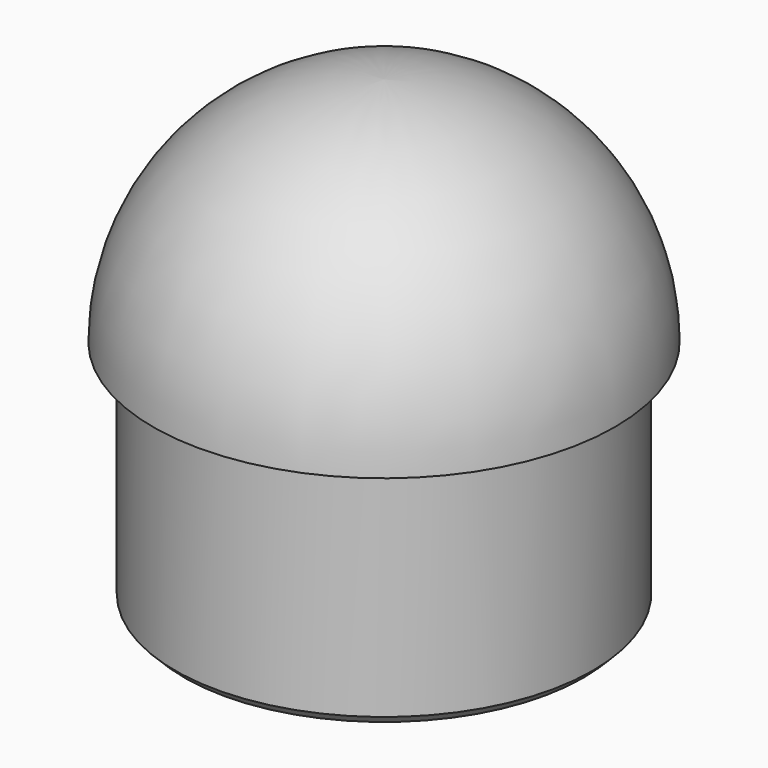
from build123d import *

# Parameters (mm, degrees)
F0_R     = 12.5
F1_DEPTH = 12.5
F2_R     = 12.49999
F3_R     = 11.3
F4_DEPTH = 12.5
F5_SIZE  = 0.5


# Not quite as in the source:
# - a fillet or chamfer is up to 0.001 mm smaller than in the source, because OpenCascade refuses the exact size


with BuildPart() as f1:
    # F0 (on Top) → F1 (new body)
    with BuildSketch(Plane.XY):
        Circle(F0_R)
    extrude(amount=F1_DEPTH)

    # F2 (radius 12.5 in the source; OpenCascade refuses exactly that, so slightly less here)
    f2_edges = [f1.edges().sort_by_distance(p)[0] for p in [
        (-12.5, 0, 12.5),
    ]]
    fillet(f2_edges, radius=F2_R)

    # F3 (on Top) → F4 (join)
    with BuildSketch(Plane.XY):
        Circle(F3_R)
    extrude(amount=-F4_DEPTH)

    # F5
    f5_edges = [f1.edges().sort_by_distance(p)[0] for p in [
        (-11.3, 0, -12.5),
    ]]
    chamfer(f5_edges, length=F5_SIZE)


solid = f1.part
